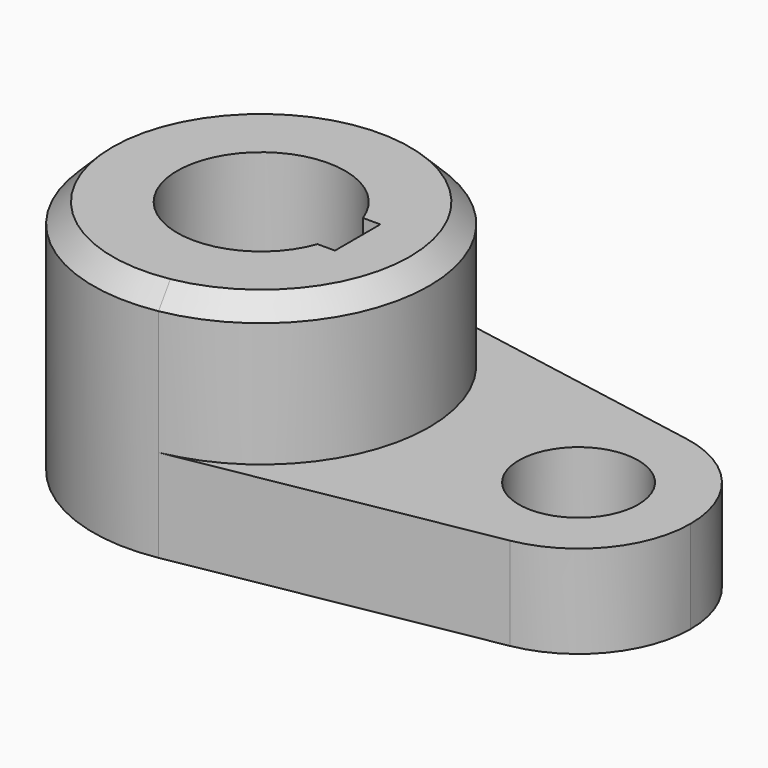
from build123d import *

# Parameters (mm, degrees)
F0_R     = 10.16
F1_DEPTH = 15.7734
F3_DEPTH = 24.4602
F4_SIZE  = 3.302


with BuildPart() as f1:
    # F0 (on Top) → F1 (new body)
    with BuildSketch(Plane.XY):
        with BuildLine():
            ThreePointArc((5.0426470588, -28.1265414802), (21.9160245563, -18.3362616868), (28.575, 0))
            ThreePointArc((28.575, 0), (21.9160245563, 18.3362616868), (5.0426470588, 28.1265414802))
            ThreePointArc((5.0426470588, 28.1265414802), (-28.575, 0), (5.0426470588, -28.1265414802))
        make_face()
        with BuildLine():
            ThreePointArc((-13.4477648793, 4.826), (0, 14.2875), (13.4477648793, 4.826))
            Line((13.4477648793, 4.826), (16.4084, 4.826))
            Line((16.4084, 4.826), (16.4084, -4.826))
            Line((16.4084, -4.826), (13.4477648793, -4.826))
            ThreePointArc((13.4477648793, -4.826), (0, -14.2875), (-13.4477648793, -4.826))
            Line((-13.4477648793, -4.826), (-16.4084, -4.826))
            Line((-16.4084, -4.826), (-16.4084, 4.826))
            Line((-16.4084, 4.826), (-13.4477648793, 4.826))
        make_face(mode=Mode.SUBTRACT)
        with BuildLine():
            ThreePointArc((5.0426470588, 28.1265414802), (21.9160245563, 18.3362616868), (28.575, 0))
            ThreePointArc((28.575, 0), (21.9160245563, -18.3362616868), (5.0426470588, -28.1265414802))
            Line((5.0426470588, -28.1265414802), (57.3367647059, -18.7510276535))
            ThreePointArc((57.3367647059, -18.7510276535), (34.925, 0), (57.3367647059, 18.7510276535))
            Line((57.3367647059, 18.7510276535), (5.0426470588, 28.1265414802))
        make_face()
        with BuildLine():
            ThreePointArc((73.025, 0), (68.5856830375, 12.2241744579), (57.3367647059, 18.7510276535))
            ThreePointArc((57.3367647059, 18.7510276535), (34.925, 0), (57.3367647059, -18.7510276535))
            ThreePointArc((57.3367647059, -18.7510276535), (68.5856830375, -12.2241744579), (73.025, 0))
        make_face()
        with Locations((53.975, 0)):
            Circle(F0_R, mode=Mode.SUBTRACT)
        with BuildLine():
            ThreePointArc((-13.4477648793, -4.826), (-14.2875, 0), (-13.4477648793, 4.826))
            Line((-13.4477648793, 4.826), (-16.4084, 4.826))
            Line((-16.4084, 4.826), (-16.4084, -4.826))
            Line((-16.4084, -4.826), (-13.4477648793, -4.826))
        make_face()
    extrude(amount=F1_DEPTH)

    # F2 (on face) → F3 (join)
    with BuildSketch(Plane.XY.offset(15.7734)):
        with BuildLine():
            ThreePointArc((5.0426470588, -28.1265414802), (21.9160245563, -18.3362616868), (28.575, 0))
            ThreePointArc((28.575, 0), (21.9160245563, 18.3362616868), (5.0426470588, 28.1265414802))
            ThreePointArc((5.0426470588, 28.1265414802), (-28.575, 0), (5.0426470588, -28.1265414802))
        make_face()
        with BuildLine():
            ThreePointArc((13.4477648793, -4.826), (-14.2875, 0), (13.4477648793, 4.826))
            Line((13.4477648793, 4.826), (16.4084, 4.826))
            Line((16.4084, 4.826), (16.4084, -4.826))
            Line((16.4084, -4.826), (13.4477648793, -4.826))
        make_face(mode=Mode.SUBTRACT)
    extrude(amount=F3_DEPTH)

    # F4
    f4_edges = [f1.edges().sort_by_distance(p)[0] for p in [
        (-5.042647, 28.126541, 40.2336),
    ]]
    chamfer(f4_edges, length=F4_SIZE)


solid = f1.part
